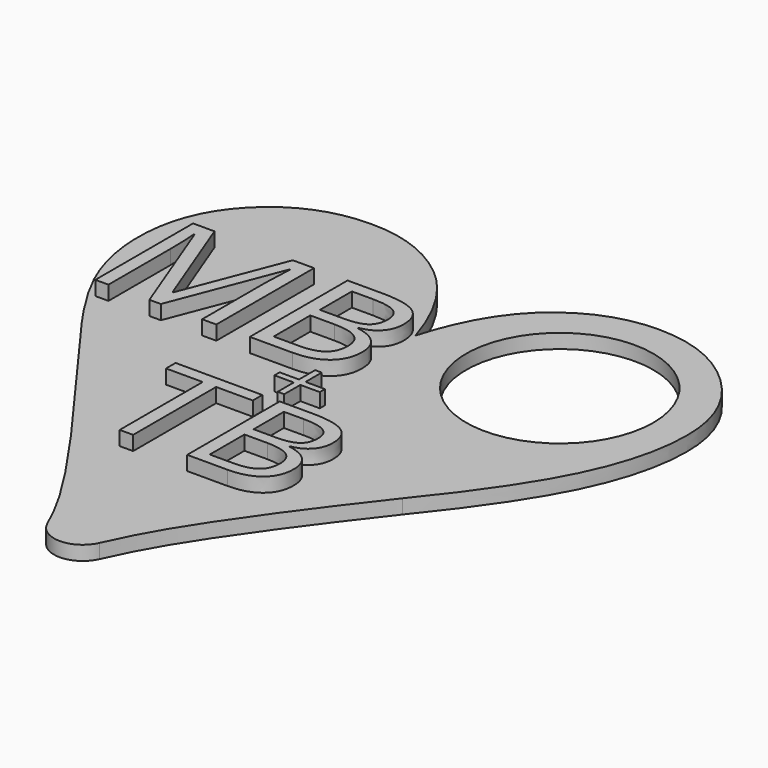
from build123d import *

# Parameters (mm, degrees)
F0_TEXT_SIZE   = 77.0513485703
F1_DEPTH       = 1
F2_TEXT_SIZE   = 11.3362220064
F2_TEXT_SIZE_2 = 6.7648788293
F2_TEXT_SIZE_3 = 11.9683901883
F3_DEPTH       = 1
F4_R           = 6.5436563848
F5_DEPTH       = 25
F6_R           = 2


# Not quite as in the source:
# - Text() gives the source's letters only with a copy of the font that has no kerning and outlines rounded to 1/6400 em; it was checked with that copy


with BuildPart() as f1:
    # F0 (on Top) → F1 (new body)
    with BuildSketch(Plane.XY):
        with Locations((-46.724419344, 0)):
            Text('♥', F0_TEXT_SIZE, font='Tinos', font_style=FontStyle.BOLD, text_align=(TextAlign.LEFT, TextAlign.BOTTOM))
    extrude(amount=F1_DEPTH)

    # F2 (on face) → F3 (join)
    with BuildSketch(Plane.XY.offset(1)):
        with Locations((-30.8865806825, 13.8985752128)):
            Text('TB', F2_TEXT_SIZE, font='Open Sans', text_align=(TextAlign.LEFT, TextAlign.BOTTOM))
        with Locations((-26.001051066, 22.0606550574)):
            Text('+', F2_TEXT_SIZE_2, font='Open Sans', text_align=(TextAlign.LEFT, TextAlign.BOTTOM))
        with Locations((-41.5268912911, 26.9313678145)):
            Text('MB', F2_TEXT_SIZE_3, font='Open Sans', text_align=(TextAlign.LEFT, TextAlign.BOTTOM))
    extrude(amount=F3_DEPTH)

    # F4 (on face) → F5 (cut)
    with BuildSketch(Plane.XY.offset(1)):
        with Locations((-13.73818703, 34.2711098492)):
            Circle(F4_R)
    extrude(amount=-F5_DEPTH, mode=Mode.SUBTRACT)

    # F6
    f6_edges = [f1.edges().sort_by_distance(p)[0] for p in [
        (-23.777565, -0.866828, 0.5),
    ]]
    fillet(f6_edges, radius=F6_R)


solid = f1.part
